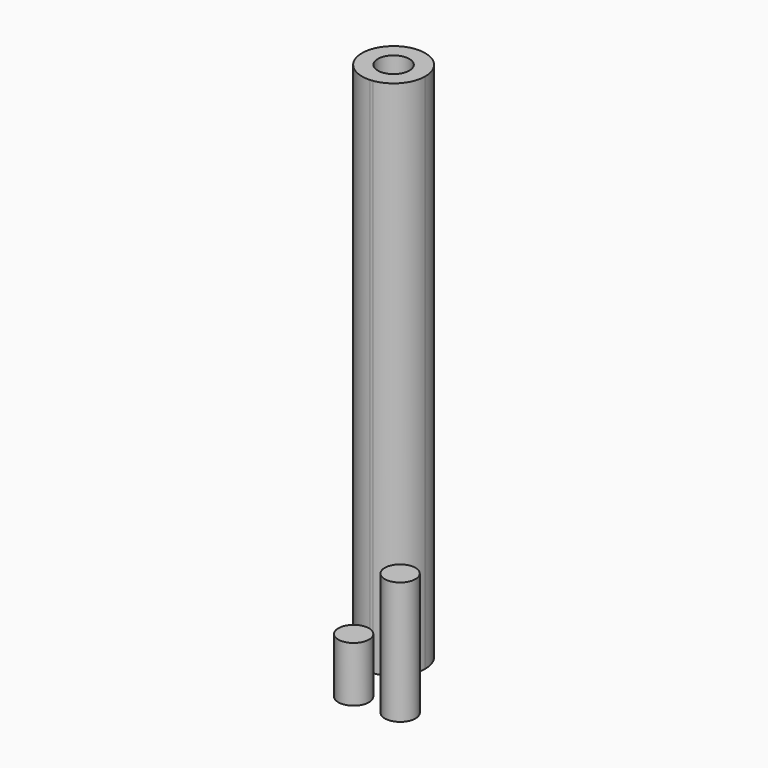
from build123d import *

# Parameters (mm, degrees)
F4_DEPTH = 170
F0_R     = 5
F5_DEPTH = 40
F6_D     = 10.3
F6_DEPTH = 23
F6_TIP   = 3.094432188
F1_DEPTH = 18
F3_D     = 10.3
F3_DEPTH = 23
F3_TIP   = 3.094432188


# Not quite as in the source:
# - a feature names something its author has since deleted; it is built from what else it names


with BuildPart() as f4:
    # F0 (on Top) → F4 (new body)
    with BuildSketch(Plane.XY):
        with BuildLine():
            ThreePointArc((1.459339769, -10.1960937343), (7.7820691214, -6.7475477167), (10.3, 0))
            ThreePointArc((10.3, 0), (-3.1805785381, 9.7966279996), (-8.335712653, -6.0502805363))
            ThreePointArc((-8.335712653, -6.0502805363), (-4.4053069437, -9.3103851012), (0.6079003247, -10.2820453799))
            ThreePointArc((0.6079003247, -10.2820453799), (1.0317778037, -10.2208202439), (1.459339769, -10.1960937343))
        make_face()
        with BuildLine():
            ThreePointArc((-6.950166537, -5.9466386188), (-7.3749932213, -5.9984609008), (-7.8016059813, -6.0325902644))
            ThreePointArc((-7.8016059813, -6.0325902644), (-7.3777285024, -5.9713651284), (-6.950166537, -5.9466386188))
        make_face(mode=Mode.SUBTRACT)
    extrude(amount=F4_DEPTH)

    # F6
    with Locations(Plane(origin=(0, 0, 0), x_dir=(1, 0, 0), z_dir=(0, 0, -1))):
        with Locations((0, 0)):
            Hole(F6_D / 2, depth=F6_DEPTH)
            with Locations((0, 0, -(F6_DEPTH + F6_TIP / 2))):  # 118° drill point
                Cone(0, F6_D / 2, F6_TIP, mode=Mode.SUBTRACT)

    # F3
    with Locations(Plane.XY.offset(170)):
        with Locations((0, 0)):
            Hole(F3_D / 2, depth=F3_DEPTH)
            with Locations((0, 0, -(F3_DEPTH + F3_TIP / 2))):  # 118° drill point
                Cone(0, F3_D / 2, F3_TIP, mode=Mode.SUBTRACT)


with BuildPart() as f5:
    # F0 (on Top) → F5 (new body)
    with BuildSketch(Plane.XY):
        with Locations((20.4564929008, -22.9047387838)):
            Circle(F0_R)
    extrude(amount=F5_DEPTH)


with BuildPart() as f1:
    # F0 (on Top) → F1 (new body)
    with BuildSketch(Plane.XY):
        with Locations((5.6373359263, -23.3221485403)):
            Circle(F0_R)
    extrude(amount=F1_DEPTH)


solid = Compound([f4.part, f5.part, f1.part])
